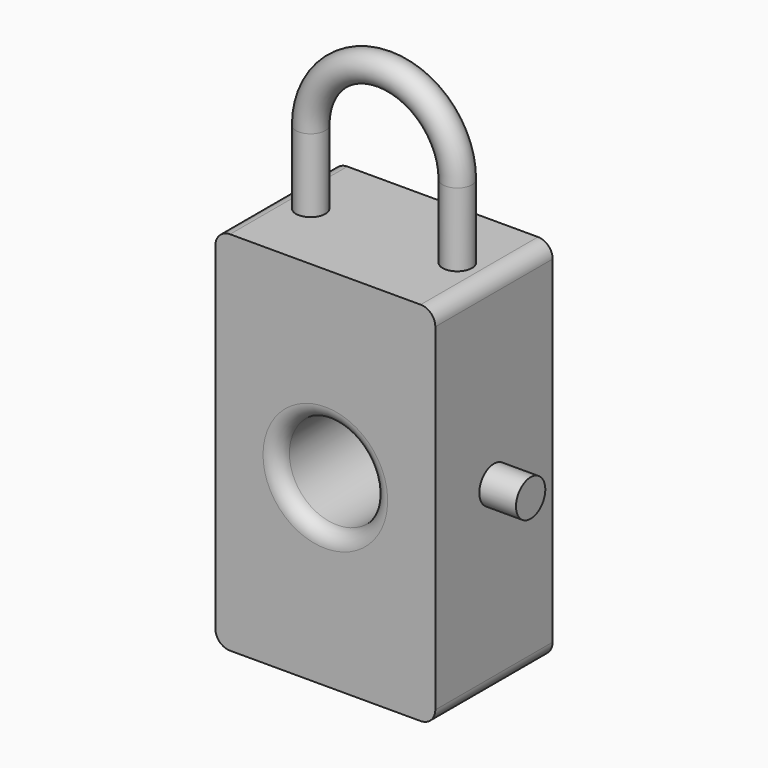
from build123d import *

# Parameters (mm, degrees)
F0_W     = 150
F0_H     = 100
F1_DEPTH = 250
F2_R     = 32.5
F3_DEPTH = 100.001
F4_R     = 10
F5_R     = 12.5
F6_DEPTH = 25
F7_R     = 10


# Not quite as in the source:
# - a pattern or mirror of a feature is missing from the dataset's text; its kind, count and spacing are read off the source's solid


with BuildPart() as f1:
    # F0 (on Top) → F1 (new body)
    with BuildSketch(Plane.XY):
        Rectangle(F0_W, F0_H)
    extrude(amount=F1_DEPTH)

    # F2 (on face) → F3 (cut, through all)
    with BuildSketch(Plane(origin=(0, 50, 0), x_dir=(-1, 0, 0), z_dir=(0, 1, 0))):
        with Locations((0, 125)):
            Circle(F2_R)
    extrude(amount=-F3_DEPTH, mode=Mode.SUBTRACT)

    # F4
    f4_edges = [f1.edges().sort_by_distance(p)[0] for p in [
        (-75, 0, 250),
        (75, 0, 250),
        (75, 0, 0),
        (-75, 0, 0),
        (32.5, -50, 125),
        (32.5, 50, 125),
    ]]
    fillet(f4_edges, radius=F4_R)

    # F5 (on face) → F6 (join)
    with BuildSketch(Plane(origin=(-75, 0, 0), x_dir=(0, -1, 0), z_dir=(-1, 0, 0))):
        with Locations((0, 125)):
            Circle(F5_R)
    f6 = extrude(amount=F6_DEPTH)

    # F6_copies: F6 across plane
    add(f6.mirror(Plane(origin=(0, 0, 0), x_dir=(0, 0, 1), z_dir=(1, 0, 0))))

    # F9: sweep along a path in F8
    with BuildLine(Plane.XZ) as f9_path:
        Line((-50, 250), (-50, 300))
        ThreePointArc((-50, 300), (0, 350), (50, 300))
        Line((50, 300), (50, 250))
    # F7 (on face) → F9 (sweep)
    with BuildSketch(Plane.XY.offset(250)):
        with Locations((50, 0)):
            Circle(F7_R)
    sweep(path=f9_path.line)


solid = f1.part
